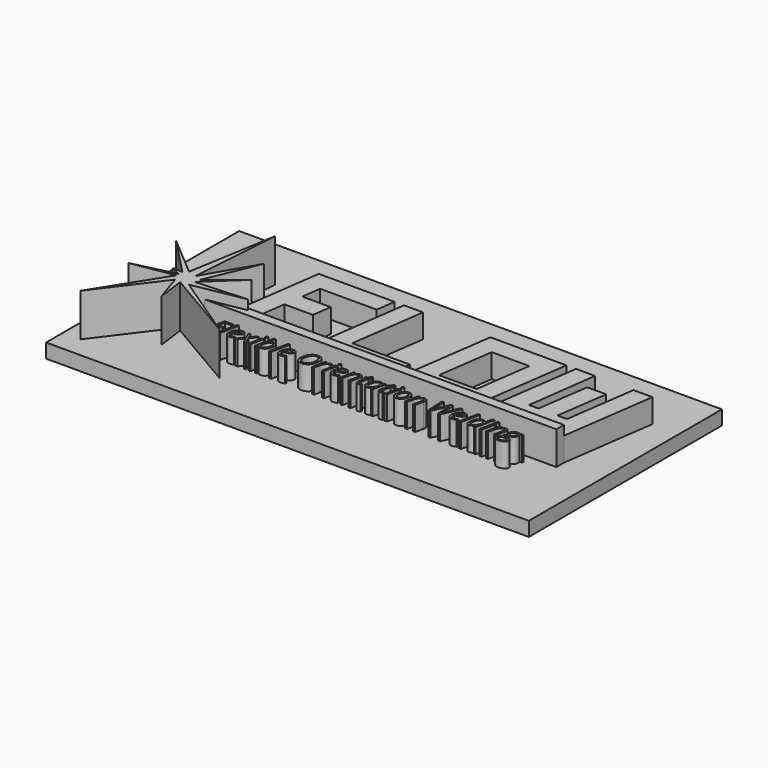
from build123d import *

# Parameters (mm, degrees)
F1_DEPTH      = 5
F3_DEPTH      = 5
F3_DEPTH_BACK = 4
F4_DEPTH      = 2
F5_TEXT_SIZE  = 5.2210447999
F6_DEPTH      = 5
F7_W          = 101.6
F7_H          = 50.8
F8_DEPTH      = 3


# Not quite as in the source:
# - Text() gives the source's letters only with a copy of the font that has no kerning and outlines rounded to 1/6400 em; it was checked with that copy


with BuildPart() as f1:
    # F0 (on Top) → F1 (new body)
    with BuildSketch(Plane.XY):
        Polygon((-14.9211019281, 7.7332906657), (65.0788980719, 7.7332906657), (65.0788980719, 9.7332906657), (48.9913015575, 9.7332906657), (46.9716464125, 9.7332906657), (30.9716464125, 9.7332906657), (28.9519912675, 9.7332906657), (12.7947501072, 9.7332906657), (-1.0969720028, 9.7332906657), (-5.1362822928, 9.7332906657), (-14.9211019281, 9.7332906657), align=None)
        Polygon((48.9913015575, 9.7332906657), (65.0788980719, 9.7332906657), (67.8623600911, 29.5386520406), (63.8623600911, 29.5386520406), (61.7747635767, 14.6846310095), (59.7747635767, 14.6846310095), (61.3056676873, 25.5775797656), (57.3056676873, 25.5775797656), (55.7747635767, 14.6846310095), (53.7747635767, 14.6846310095), (55.7747635767, 29.5386520406), (51.7747635767, 29.5386520406), align=None)
        Polygon((-2.3528202736, 29.5386520406), (-5.1362822928, 9.7332906657), (-1.0969720028, 9.7332906657), (0, 17.5386520406), (6, 17.5386520406), (6.5621633388, 21.5386520406), (0.5621633388, 21.5386520406), (1.1243266776, 25.5386520406), (13.0160487875, 25.5386520406), (13.5782121264, 29.5386520406), align=None)
        Polygon((30.9716464125, 9.7332906657), (46.9716464125, 9.7332906657), (49.7551084317, 29.5386520406), (33.7551084317, 29.5386520406), align=None)
        Polygon((35.5731200414, 13.7332906657), (37.232255383, 25.5386520406), (45.1536348028, 25.5386520406), (43.4944994612, 13.7332906657), align=None, mode=Mode.SUBTRACT)
        Polygon((15.5782121264, 29.5386520406), (12.7947501072, 9.7332906657), (28.9519912675, 9.7332906657), (29.5086836713, 13.6943629407), (17.351442511, 13.6943629407), (19.5782121264, 29.5386520406), align=None)
    extrude(amount=-F1_DEPTH)

    # F2 (on Top) → F3 (join, two sides)
    with BuildSketch(Plane.XY) as f3_sk:
        Polygon((-11.5529159084, 29.4768735766), (-14.6968239223, 10.8353141016), (-23.3481135219, 18.1982964277), (-15.5094880611, 10.0823417306), (-17.6261924207, 10.0823417306), (-15.5411055312, 9.1498149559), (-24.3808161467, 7.0176762529), (-15.5094880611, 8.5154615811), (-24.3808161467, -5.6301401928), (-14.7253191099, 7.2073759511), (-12.7674294636, 1.1343557853), (-13.5238878429, 7.0176762529), (2.057808917, -2.1060223226), (-11.8391855973, 7.2073759511), (-0.9500859305, 9.1735832393), (-11.7124812678, 8.5638118908), (-4.8603499308, 14.9637814611), (-11.5529159084, 9.4577573827), (-6.8154814653, 20.7539796829), (-12.9108829424, 10.2713555098), align=None)
    extrude(amount=-F3_DEPTH)
    extrude(f3_sk.sketch, amount=F3_DEPTH_BACK)

    # F0 (on Top) → F4 (join)
    with BuildSketch(Plane.XY):
        Polygon((-14.9211019281, 7.7332906657), (65.0788980719, 7.7332906657), (65.0788980719, 9.7332906657), (48.9913015575, 9.7332906657), (46.9716464125, 9.7332906657), (30.9716464125, 9.7332906657), (28.9519912675, 9.7332906657), (12.7947501072, 9.7332906657), (-1.0969720028, 9.7332906657), (-5.1362822928, 9.7332906657), (-14.9211019281, 9.7332906657), align=None)
    extrude(amount=F4_DEPTH)


with BuildPart() as f6:
    # F5 (on face) → F6 (new body)
    with BuildSketch(Plane.XY):
        with Locations((-4.9075558782, 2.9703490436)):
            Text('Flexible Orientation Welding', F5_TEXT_SIZE, font='Open Sans', font_style=FontStyle.ITALIC, text_align=(TextAlign.LEFT, TextAlign.BOTTOM))
    extrude(amount=-F6_DEPTH)


with BuildPart() as f8:
    # F7 (on face) → F8 (new body)
    with BuildSketch(Plane(origin=(0, 0, -5), x_dir=(1, 0, 0), z_dir=(0, 0, -1))):
        with Locations((22.6944740862, -15.3771487772)):
            Rectangle(F7_W, F7_H)
    extrude(amount=F8_DEPTH)


solid = Compound([f1.part, f6.part, f8.part])
